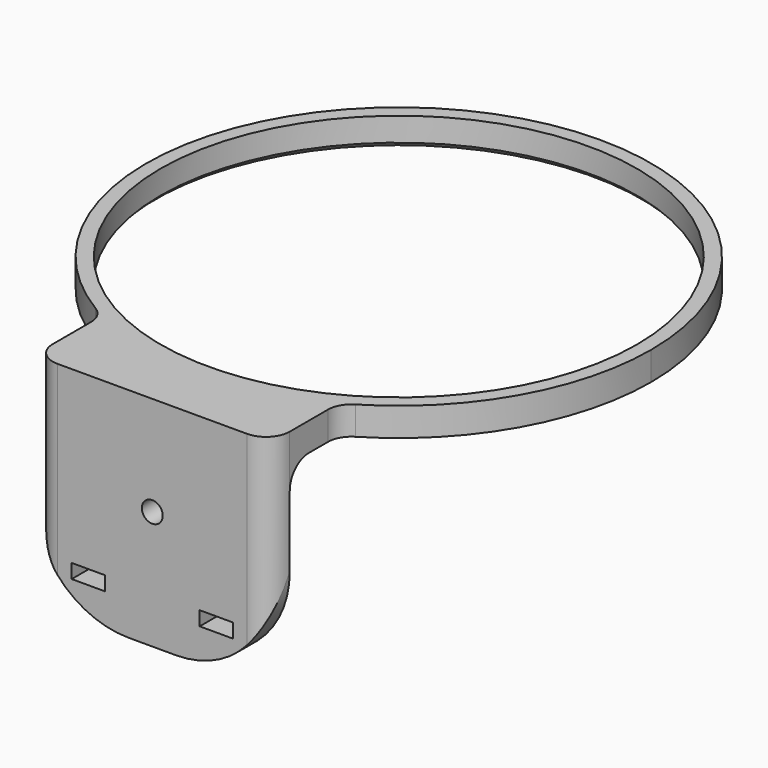
from build123d import *

# Parameters (mm, degrees)
F0_R        = 50.25
F1_DEPTH    = 6
F2_DEPTH    = 40
F4_D        = 4.4
F3_W        = 7
F3_H        = 3
F5_DEPTH    = 25
F6_R        = 5
F7_R        = 20
F8_T1_DEPTH = 59.75
F9_SIZE     = 1


# Not quite as in the source:
# - a fillet or chamfer that OpenCascade refuses, or shapes differently, is made with other operations: its cross-section is extruded or revolved along the edge and cut away or added


with BuildPart() as f1:
    # F0 (on Top) → F1 (new body)
    with BuildSketch(Plane.XY):
        with BuildLine():
            ThreePointArc((25, -47.0166194021), (45.6443452138, -27.4254671792), (53.25, 0))
            ThreePointArc((53.25, 0), (-27.4254671792, 45.6443452138), (-25, -47.0166194021))
            ThreePointArc((-25, -47.0166194021), (0, -53.25), (25, -47.0166194021))
        make_face()
        Circle(F0_R, mode=Mode.SUBTRACT)
        with BuildLine():
            ThreePointArc((25, -47.0166194021), (0, -53.25), (-25, -47.0166194021))
            Line((-25, -47.0166194021), (-25, -60))
            Line((-25, -60), (25, -60))
            Line((25, -60), (25, -47.0166194021))
        make_face()
        Polygon((25, -60), (-25, -60), (-25, -65), (0, -65), (25, -65), align=None)
    extrude(amount=F1_DEPTH)

    # F0 (on Top) → F2 (join)
    with BuildSketch(Plane.XY):
        Polygon((25, -60), (-25, -60), (-25, -65), (0, -65), (25, -65), align=None)
    extrude(amount=-F2_DEPTH)

    # F4 (through all)
    with Locations(Plane(origin=(0, -60, 0), x_dir=(-1, 0, 0), z_dir=(0, 1, 0))):
        with Locations((0, -15)):
            Hole(F4_D / 2)

    # F3 (on face) → F5 (cut)
    with BuildSketch(Plane(origin=(0, -60, 0), x_dir=(-1, 0, 0), z_dir=(0, 1, 0))):
        with Locations((-13.5, -31.5)):
            Rectangle(F3_W, F3_H)
        with Locations((13.5, -31.5)):
            Rectangle(F3_W, F3_H)
    extrude(amount=-F5_DEPTH, mode=Mode.SUBTRACT)

    # F6
    f6_edges = [f1.edges().sort_by_distance(p)[0] for p in [
        (-25, -47.016619, 3),
        (25, -47.016619, 3),
        (0, -60, 0),
    ]]
    fillet(f6_edges, radius=F6_R)

    # F7
    f7_edges = [f1.edges().sort_by_distance(p)[0] for p in [
        (25, -62.5, -40),
        (-25, -62.5, -40),
    ]]
    fillet(f7_edges, radius=F7_R)

    # F8: fillet of radius 5 on 2 edges, made by hand

    # F8_s2 → F8_t1 (cut)
    with BuildSketch(Plane.XY.offset(-41.25)):
        with BuildLine():
            ThreePointArc((25, -60), (23.5355339059, -63.5355339059), (20, -65))
            Line((20, -65), (25, -65))
            Line((25, -65), (25, -60))
        make_face()
        with BuildLine():
            ThreePointArc((-20, -65), (-23.5355339059, -63.5355339059), (-25, -60))
            Line((-25, -60), (-25, -65))
            Line((-25, -65), (-20, -65))
        make_face()
    extrude(amount=F8_T1_DEPTH, mode=Mode.SUBTRACT)

    # F9
    f9_edges = [f1.edges().sort_by_distance(p)[0] for p in [
        (-50.25, 0, 0),
    ]]
    chamfer(f9_edges, length=F9_SIZE)


solid = f1.part
